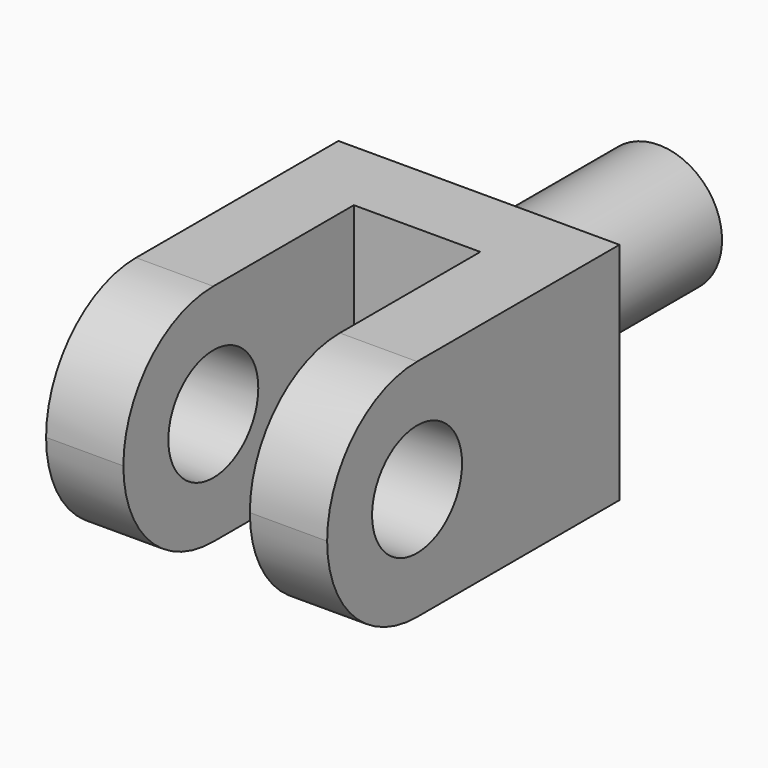
from build123d import *

# Parameters (mm, degrees)
F1_DEPTH = 812.8
F2_W     = 457.2
F2_H     = 812.8
F3_DEPTH = 812.8
F4_R     = 406.4
F6_DEPTH = 812.8
F7_R     = 406.39999
F8_R     = 203.2
F9_DEPTH = 1016.001


# Not quite as in the source:
# - a fillet or chamfer is up to 0.001 mm smaller than in the source, because OpenCascade refuses the exact size


with BuildPart() as f1:
    # F0 (on Top) → F1 (new body)
    with BuildSketch(Plane.XY):
        Polygon((0, 983.1417049408), (0, -58.2582950592), (279.4, -58.2582950592), (279.4, 1262.5417049408), (-736.6, 1262.5417049408), (-736.6, -58.2582950592), (-457.2, -58.2582950592), (-457.2, 983.1417049408), align=None)
    extrude(amount=F1_DEPTH)

    # F2 (on face) → F3 (join)
    with BuildSketch(Plane.XY.offset(812.8)):
        with Locations((-228.6, 1668.9417049408)):
            Rectangle(F2_W, F2_H)
    extrude(amount=-F3_DEPTH)

    # F4
    f4_edges = [f1.edges().sort_by_distance(p)[0] for p in [
        (139.7, -58.258295, 812.8),
        (-596.9, -58.258295, 812.8),
    ]]
    fillet(f4_edges, radius=F4_R)

    # F5 (on face) → F6 (cut)
    with BuildSketch(Plane(origin=(0, 2075.3417049408, 0), x_dir=(-1, 0, 0), z_dir=(0, 1, 0))):
        with BuildLine():
            ThreePointArc((0, 406.4), (228.6, 635), (457.2, 406.4))
            Line((457.2, 406.4), (457.2, 812.8))
            Line((457.2, 812.8), (0, 812.8))
            Line((0, 812.8), (0, 406.4))
        make_face()
        with BuildLine():
            Line((457.2, 0), (457.2, 406.4))
            ThreePointArc((457.2, 406.4), (228.6, 177.8), (0, 406.4))
            Line((0, 406.4), (0, 0))
            Line((0, 0), (457.2, 0))
        make_face()
    extrude(amount=-F6_DEPTH, mode=Mode.SUBTRACT)

    # F7 (radius 406.4 in the source; OpenCascade refuses exactly that, so slightly less here)
    f7_edges = [f1.edges().sort_by_distance(p)[0] for p in [
        (139.7, -58.258295, 0),
        (-596.9, -58.258295, 0),
    ]]
    fillet(f7_edges, radius=F7_R)

    # F8 (on face) → F9 (cut, through all)
    with BuildSketch(Plane.YZ.offset(279.4)):
        with Locations((348.1417049408, 406.4)):
            Circle(F8_R)
    extrude(amount=-F9_DEPTH, mode=Mode.SUBTRACT)


solid = f1.part
